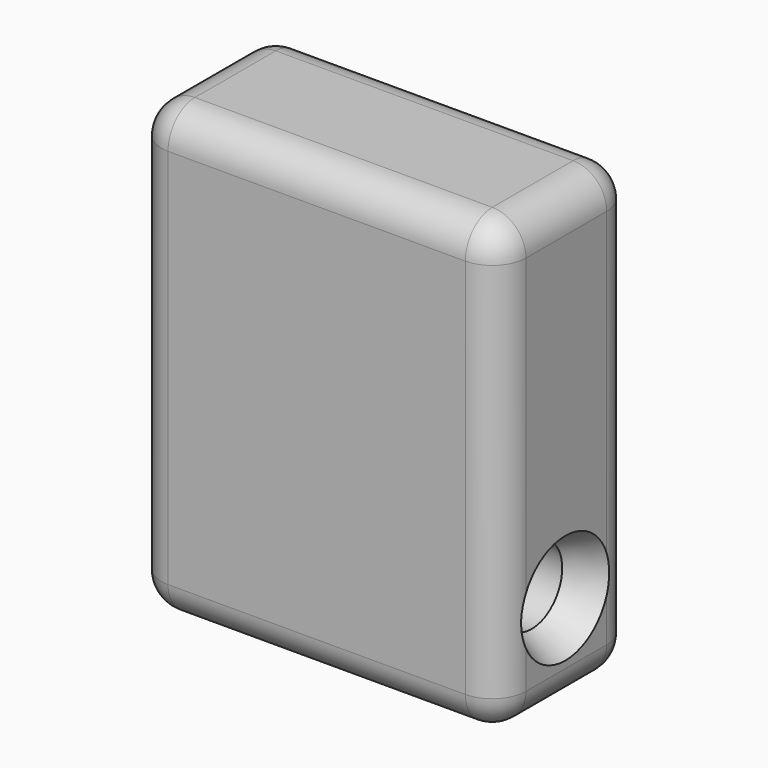
from build123d import *

# Parameters (mm, degrees)
F0_W     = 65
F0_H     = 80
F1_DEPTH = 30
F2_R     = 6.7948556495
F3_DEPTH = 65
F4_R     = 6
F6_T     = -2


# Not quite as in the source:
# - a fillet or chamfer that OpenCascade refuses, or shapes differently, is made with other operations: its cross-section is extruded or revolved along the edge and cut away or added
# - a shell that OpenCascade refuses in one call is made with other operations: the cavity is built on its own and cut out


with BuildPart() as f1:
    # F0 (on Front) → F1 (new body)
    with BuildSketch(Plane.XZ):
        with Locations((32.5, 40)):
            Rectangle(F0_W, F0_H)
    extrude(amount=-F1_DEPTH)

    # F2 (on Right) → F3 (cut, through all)
    with BuildSketch(Plane.YZ):
        with Locations((14.7847002372, 17.048144713)):
            Circle(F2_R)
    extrude(amount=F3_DEPTH, mode=Mode.SUBTRACT)

    # F4
    f4_edges = [f1.edges().sort_by_distance(p)[0] for p in [
        (65, 15, 80),
        (32.5, 0, 80),
        (65, 0, 40),
        (32.5, 0, 0),
        (0, 0, 40),
        (0, 15, 0),
        (0, 30, 40),
        (32.5, 30, 0),
        (65, 15, 0),
        (0, 15, 80),
        (65, 30, 40),
        (32.5, 30, 80),
    ]]
    fillet(f4_edges, radius=F4_R)

    # F5: chamfer of 3 x 6 on 3 edges, made by hand

    # F5_s1 → F5_t2 (revolve, cut)
    with BuildSketch(Plane.XY.offset(17.048144713)):
        Polygon((65, 24.5795558867), (59, 21.5795558867), (65, 21.5795558867), align=None)
    revolve(axis=Axis((65, 14.7847002372, 17.048144713), (1, 0, 0)), mode=Mode.SUBTRACT)

    # F5_s3 → F5_t4 (revolve, cut)
    with BuildSketch(Plane.XY.offset(17.048144713)):
        Polygon((6, 21.5795558867), (0, 24.5795558867), (0, 21.5795558867), align=None)
    revolve(axis=Axis((0, 14.7847002372, 17.048144713), (1, 0, 0)), mode=Mode.SUBTRACT)

    # F6: a shell. OpenCascade refuses it in one call, so the cavity is built on its own and cut out:
    # the body offset inwards by the wall thickness, plus a prism from it out through each open face.
    f6_core = offset(f1.part, amount=F6_T, mode=Mode.PRIVATE)
    f6_exits = [f6_core.faces().sort_by_distance(p)[0] for p in [
        (32.5, 28, 40),
    ]]
    add(f6_core, mode=Mode.SUBTRACT)
    extrude(f6_exits, amount=-F6_T, mode=Mode.SUBTRACT)


solid = f1.part
